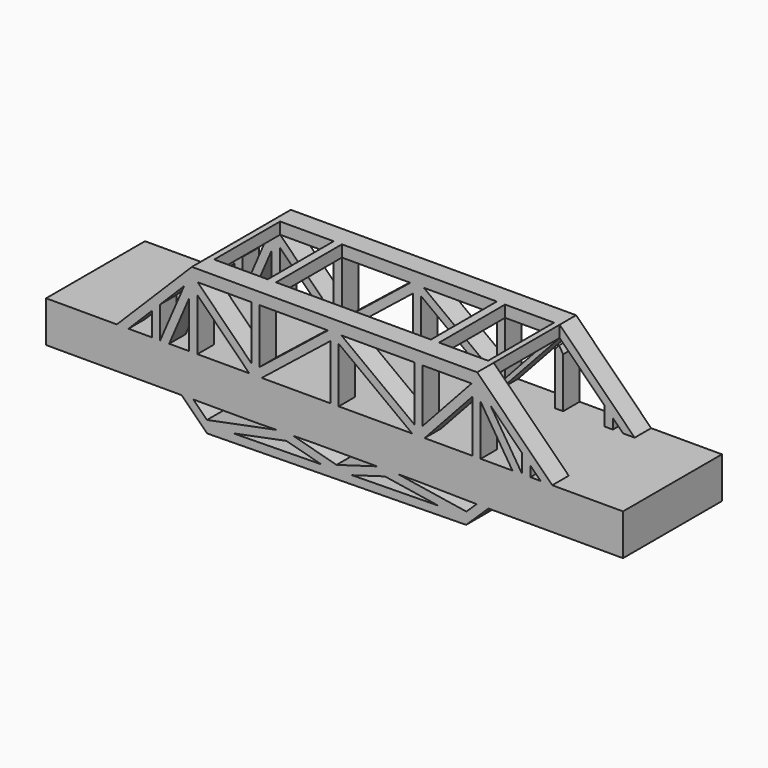
from build123d import *

# Parameters (mm, degrees)
F1_DEPTH  = 19.05
F2_DEPTH  = 19.05
F3_DEPTH  = 12.7
F4_DEPTH  = 6.35
F5_DEPTH  = 6.35
F7_DEPTH  = 6.35
F8_DEPTH  = 6.35
F11_DEPTH = 25.4
F12_DEPTH = 25.4
F6_W      = 1.7239038059
F6_H      = 3.5921024484
F6_W_2    = 1.7933621035
F13_DEPTH = 38.1
F14_DEPTH = 6.35


# Not quite as in the source:
# - a feature names something its author has since deleted; it is built from what else it names


with BuildPart() as f1:
    # F0 (on Front) → F1 (new body)
    with BuildSketch(Plane.XZ):
        Polygon((-75.3014223417, -8.4543359262), (-75.3014223417, -1.435443759), (-78.8935247901, -1.435443759), (-100.7014223417, -1.435443759), (-100.7014223417, -14.135443759), (-75.3014223417, -14.135443759), align=None)
    extrude(amount=-F1_DEPTH)

    # F0 (on Front) → F2 (join)
    with BuildSketch(Plane.XZ):
        Polygon((-68.0739664064, -1.435443759), (-75.3014223417, -1.435443759), (-75.3014223417, -8.4543359262), (-75.3014223417, -14.135443759), (-58.9322418971, -14.135443759), (-55.3401394486, -14.135443759), (-55.3401394486, -1.435443759), (-56.6101394486, -1.435443759), (-62.7698475104, -1.435443759), (-64.1519069584, -1.435443759), (-65.5339664064, -1.435443759), align=None)
        Polygon((-55.3401394486, -1.435443759), (-55.3401394486, -14.135443759), (-36.2901394486, -14.135443759), (-36.2901394486, -1.435443759), (-38.0835015521, -1.435443759), (-54.0701394486, -1.435443759), align=None)
        Polygon((-34.2535879934, -1.435443759), (-36.2901394486, -1.435443759), (-36.2901394486, -14.135443759), (-29.5884479715, -14.0381948012), (-24.5761177188, -13.9654603438), (-18.1276498189, -13.8718859402), (-18.1276498189, -1.435443759), align=None)
    extrude(amount=-F2_DEPTH)



with BuildPart() as f1b:
    # F0 (on Front) → F1, piece 2 (new body)
    with BuildSketch(Plane.XZ):
        Polygon((77.0985776583, -1.435443759), (55.2906801068, -1.435443759), (51.6985776583, -1.435443759), (48.562251594, -1.435443759), (46.022251594, -1.435443759), (44.5195358117, -1.435443759), (43.0168200294, -1.435443759), (33.2472785554, -1.435443759), (31.9772785554, -1.435443759), (31.9772785554, -14.135443759), (35.6239399467, -14.135443759), (77.0985776583, -14.135443759), align=None)
    extrude(amount=-F1_DEPTH)

    # F0 (on Front) → F2, piece 2 (join)
    with BuildSketch(Plane.XZ):
        Polygon((14.2324982387, -13.8718859402), (14.2324982387, -1.435443759), (12.1164883202, -1.435443759), (-5.4276498189, -1.435443759), (-5.4276498189, -13.8718859402), (1.2740385811, -13.8718859402), (7.7840224387, -13.8718859402), align=None)
        Polygon((15.9564020446, -1.435443759), (14.2324982387, -1.435443759), (14.2324982387, -13.8718859402), (31.9772785554, -14.135443759), (31.9772785554, -1.435443759), (30.7072785554, -1.435443759), align=None)
        Polygon((77.0985776583, -1.435443759), (55.2906801068, -1.435443759), (51.6985776583, -1.435443759), (48.562251594, -1.435443759), (46.022251594, -1.435443759), (44.5195358117, -1.435443759), (43.0168200294, -1.435443759), (33.2472785554, -1.435443759), (31.9772785554, -1.435443759), (31.9772785554, -14.135443759), (35.6239399467, -14.135443759), (77.0985776583, -14.135443759), align=None)
    extrude(amount=-F2_DEPTH)


with BuildPart() as f1_1:
    add(f1.part)
    # F3 (add, through all): a face of the model
    f3_faces = [f1b.part.faces().sort_by_distance(p)[0] for p in [
        (-5.4276498189, 9.525, -7.6536648496),
    ]]

    add(f1b.part)  # F3 merges F1b
    extrude(f3_faces, amount=F3_DEPTH)

    # F0 (on Front) → F4 (join)
    with BuildSketch(Plane.XZ):
        Polygon((-78.8935247901, -1.435443759), (-75.3014223417, -1.435443759), (-68.0739664064, 5.7920121763), (-65.5339664064, 8.3320121763), (-58.1879977366, 15.6779808461), (-55.7665104711, 18.0994681116), (-53.9731483676, 18.0994681116), (-37.4634148507, 18.0994681116), (-36.1934148507, 18.0994681116), (-34.9234148507, 18.0994681116), (-13.8379737969, 18.0994681116), (-11.8014223417, 18.0994681116), (-9.6854124232, 18.0994681116), (12.8047038004, 18.0994681116), (14.0747038004, 18.0994681116), (15.3447038004, 18.0994681116), (30.4397619819, 18.0994681116), (32.1636657878, 18.0994681116), (36.2527101199, 14.0104237794), (46.022251594, 4.2408823054), (48.562251594, 1.7008823054), (51.6985776583, -1.435443759), (55.2906801068, -1.435443759), (32.1636657878, 21.69157056), (-55.7665104711, 21.69157056), align=None)
        Polygon((-68.0739664064, 5.7920121763), (-68.0739664064, -1.435443759), (-65.5339664064, -1.435443759), (-65.5339664064, 8.3320121763), align=None)
        Polygon((-36.1934148507, 18.0994681116), (-37.4634148507, 18.0994681116), (-37.4634148507, 1.5401106785), (-36.1934148507, 0.2662933926), align=None)
        Polygon((-34.9234148507, 18.0994681116), (-36.1934148507, 18.0994681116), (-36.1934148507, 0.2662933926), (-34.9234148507, 1.2793859922), align=None)
        Polygon((-11.7776498189, 16.4938528035), (-13.0476498189, 15.4807602039), (-13.0476498189, -1.435443759), (-11.7776498189, -1.435443759), align=None)
        Polygon((-10.5076498189, 15.5408907631), (-11.7776498189, 16.4938528035), (-11.7776498189, -1.435443759), (-10.5076498189, -1.435443759), align=None)
        Polygon((15.3447038004, 18.0994681116), (14.0747038004, 18.0994681116), (14.0747038004, 0.2707367444), (15.3447038004, 1.6543241772), align=None)
        Polygon((14.0747038004, 18.0994681116), (12.8047038004, 18.0994681116), (12.8047038004, 1.2236987848), (14.0747038004, 0.2707367444), align=None)
        Polygon((30.7072785554, -1.435443759), (31.9772785554, -1.435443759), (31.9772785554, 16.0183226994), (30.7072785554, 14.6347352666), align=None)
        Polygon((31.9772785554, 16.0183226994), (31.9772785554, -1.435443759), (33.2472785554, -1.435443759), (33.2472785554, 14.0104237794), align=None)
        Polygon((-55.3401394486, 15.8730630517), (-55.3401394486, -1.435443759), (-54.0701394486, -1.435443759), (-54.0701394486, 14.5992457658), align=None)
        Polygon((-56.6101394486, 12.9144267948), (-56.6101394486, -1.435443759), (-55.3401394486, -1.435443759), (-55.3401394486, 15.8730630517), align=None)
    extrude(amount=-F4_DEPTH)

    # F0 (on Front) → F5 (join)
    with BuildSketch(Plane.XZ):
        Polygon((-55.7665104711, 18.0994681116), (-64.1519069584, -1.435443759), (-62.7698475104, -1.435443759), (-56.6101394486, 12.9144267948), (-55.3401394486, 15.8730630517), (-54.0701394486, 14.5992457658), (-38.0835015521, -1.435443759), (-36.2901394486, -1.435443759), align=None)
        Polygon((-58.1879977366, 15.6779808461), (-65.5339664064, -1.435443759), (-64.1519069584, -1.435443759), (-55.7665104711, 18.0994681116), align=None)
        Polygon((-53.9731483676, 18.0994681116), (-55.7665104711, 18.0994681116), (-36.2901394486, -1.435443759), (-11.8014223417, 18.0994681116), (-13.8379737969, 18.0994681116), (-34.9234148507, 1.2793859922), (-36.1934148507, 0.2662933926), (-37.4634148507, 1.5401106785), align=None)
        Polygon((-11.8014223417, 18.0994681116), (-36.2901394486, -1.435443759), (-34.2535879934, -1.435443759), (-13.0476498189, 15.4807602039), (-11.7776498189, 16.4938528035), (-10.5076498189, 15.5408907631), (12.1164883202, -1.435443759), (14.2324982387, -1.435443759), align=None)
        Polygon((-9.6854124232, 18.0994681116), (-11.8014223417, 18.0994681116), (14.2324982387, -1.435443759), (32.1636657878, 18.0994681116), (30.4397619819, 18.0994681116), (15.3447038004, 1.6543241772), (14.0747038004, 0.2707367444), (12.8047038004, 1.2236987848), align=None)
    extrude(amount=-F5_DEPTH)

    # F0 (on Front) → F7 (join)
    with BuildSketch(Plane.XZ):
        Polygon((-55.3401394486, -14.135443759), (-58.9322418971, -14.135443759), (-51.0965817995, -21.9711038566), (28.7455422806, -20.8125063022), (35.6239399467, -14.135443759), (31.9772785554, -14.135443759), (28.8399389893, -17.1809513785), (27.7001179184, -18.2874091537), (20.2112810939, -18.3960804614), (-6.4368105921, -18.782773754), (-11.1798369081, -18.8516003134), (-15.855044379, -18.9194427462), (-43.0566496336, -19.3141681332), (-50.0597917346, -19.415791473), (-51.1394793261, -18.3361038815), align=None)
        Polygon((-26.606417659, -14.7384993405), (-50.0597917346, -19.415791473), (-43.0566496336, -19.3141681332), (-26.647951981, -16.0417915366), (-15.855044379, -18.9194427462), (-11.1798369081, -18.8516003134), align=None)
        Polygon((-29.5884479715, -14.0381948012), (-51.1394793261, -18.3361038815), (-50.0597917346, -19.415791473), (-26.606417659, -14.7384993405), (-11.1798369081, -18.8516003134), (3.6282092287, -14.5043621946), (27.7001179184, -18.2874091537), (28.8399389893, -17.1809513785), (7.7840224387, -13.8718859402), (1.2740385811, -13.8718859402), (-11.1963136804, -17.5328409511), (-24.5761177188, -13.9654603438), align=None)
        Polygon((3.6282092287, -14.5043621946), (-11.1798369081, -18.8516003134), (-6.4368105921, -18.782773754), (3.7125368777, -15.8032023917), (20.2112810939, -18.3960804614), (27.7001179184, -18.2874091537), align=None)
    extrude(amount=-F7_DEPTH)

    # F0 (on Front) → F8 (join)
    with BuildSketch(Plane.XZ):
        Polygon((46.022251594, -1.435443759), (48.562251594, -1.435443759), (48.562251594, 1.7008823054), (46.022251594, 4.2408823054), align=None)
    extrude(amount=-F8_DEPTH)

    # F9: F1 across face


with BuildPart() as f1_2:
    add(f1_1.part)
    add(f1_1.part.mirror(Plane(origin=(-11.8589412224, 19.05, -7.7486185811), x_dir=(-1, 0, 0), z_dir=(0, 1, 0))))

    # F10 (on face) → F11 (join, through all)
    with BuildSketch(Plane.XZ.offset(-31.75)):
        Polygon((20.248135424, -20.9358130769), (28.7455422806, -20.8125063022), (28.7086879505, -18.2727736867), (20.2112810939, -18.3960804614), align=None)
    extrude(amount=F11_DEPTH)

    # F10 (on face) → F12 (join, through all)
    with BuildSketch(Plane.XZ.offset(-31.75)):
        Polygon((-43.0566496336, -21.8544355458), (-43.0566496336, -19.3141681332), (-51.0965817995, -19.3141681332), (-51.0965817995, -19.325645402), (-51.0965817995, -21.9711038566), align=None)
    extrude(amount=F12_DEPTH)

    # F6 (on face) → F13 (join)
    with BuildSketch(Plane.XZ):
        Polygon((15.3447038004, 18.0994681116), (15.3447038004, 21.69157056), (12.8047038004, 21.69157056), (12.8047038004, 18.0994681116), (14.0747038004, 18.0994681116), align=None)
        with Locations((31.3017138849, 19.8955193358)):
            Rectangle(F6_W, F6_H)
        with Locations((-54.8698294194, 19.8955193358)):
            Rectangle(F6_W_2, F6_H)
        Polygon((-34.9234148507, 18.0994681116), (-34.9234148507, 21.69157056), (-37.4634148507, 21.69157056), (-37.4634148507, 18.0994681116), (-36.1934148507, 18.0994681116), align=None)
    extrude(amount=-F13_DEPTH)

    # F0 (on Front) → F14 (join)
    with BuildSketch(Plane.XZ):
        Polygon((32.1636657878, 18.0994681116), (14.2324982387, -1.435443759), (15.9564020446, -1.435443759), (30.7072785554, 14.6347352666), (31.9772785554, 16.0183226994), (33.2472785554, 14.0104237794), (43.0168200294, -1.435443759), (44.5195358117, -1.435443759), align=None)
        Polygon((44.5195358117, -1.435443759), (46.022251594, -1.435443759), (36.2527101199, 14.0104237794), (32.1636657878, 18.0994681116), align=None)
    extrude(amount=-F14_DEPTH)


solid = f1_2.part
